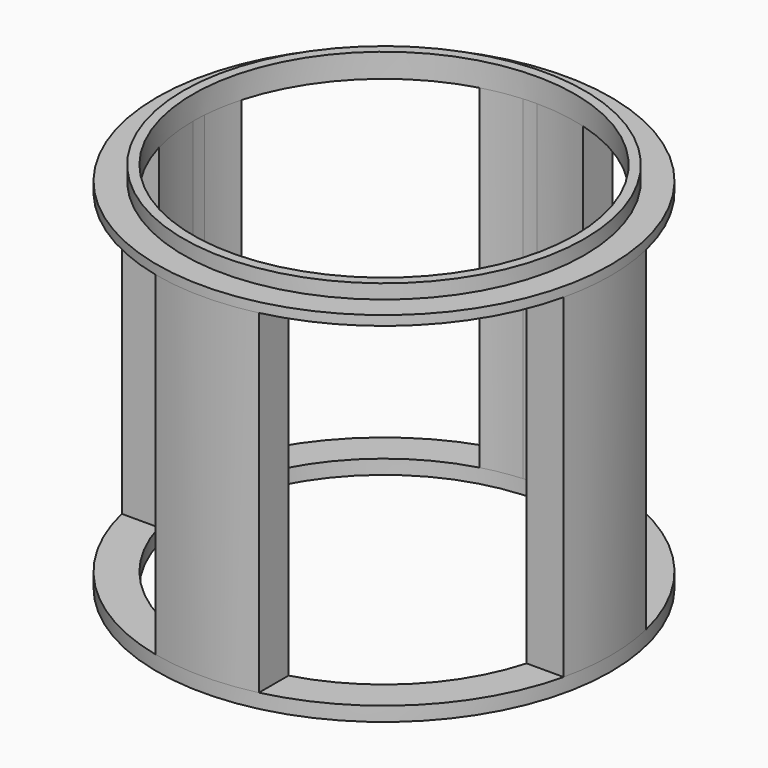
from build123d import *

# Parameters (mm, degrees)
F0_R     = 47.5
F0_R_2   = 40
F1_DEPTH = 3
F3_DEPTH = 70
F4_R     = 47.5
F4_R_2   = 40
F5_DEPTH = 2
F6_R     = 42
F6_R_2   = 40
F7_DEPTH = 3


# Not quite as in the source:
# - after a boolean that leaves OpenCascade's solid faulty, fix() repairs it


with BuildPart() as f1:
    # F0 (on Top) → F1 (new body)
    with BuildSketch(Plane.XY):
        Circle(F0_R)
        Circle(F0_R_2, mode=Mode.SUBTRACT)
    extrude(amount=F1_DEPTH)

    # F2 (on face) → F3 (join)
    with BuildSketch(Plane.XY.offset(3)):
        with BuildLine():
            Line((10.811338, 38.511232), (10.811338, 46.25327))
            ThreePointArc((10.811338, 46.25327), (0, 47.5), (-10.811338, 46.25327))
            Line((-10.811338, 46.25327), (-10.811338, 38.511232))
            ThreePointArc((-10.811338, 38.511232), (-6.865711, 39.40637), (-2.849842, 39.898351))
            ThreePointArc((-2.849842, 39.898351), (-1.425827, 39.97458), (0, 40))
            ThreePointArc((0, 40), (5.456681, 39.62606), (10.811338, 38.511232))
        make_face()
        with BuildLine():
            ThreePointArc((-39.898351, 2.849838), (-39.406371, 6.865709), (-38.511232, 10.811338))
            Line((-38.511232, 10.811338), (-46.25327, 10.811338))
            ThreePointArc((-46.25327, 10.811338), (-47.5, 0), (-46.25327, -10.811338))
            Line((-46.25327, -10.811338), (-38.511232, -10.811338))
            ThreePointArc((-38.511232, -10.811338), (-39.62606, -5.456681), (-40, 0))
            ThreePointArc((-40, 0), (-39.97458, 1.425825), (-39.898351, 2.849838))
        make_face()
        with BuildLine():
            Line((-10.811338, -38.511232), (-10.811338, -46.25327))
            ThreePointArc((-10.811338, -46.25327), (0, -47.5), (10.811338, -46.25327))
            Line((10.811338, -46.25327), (10.811338, -38.511232))
            ThreePointArc((10.811338, -38.511232), (5.456681, -39.62606), (0, -40))
            ThreePointArc((0, -40), (-5.456681, -39.62606), (-10.811338, -38.511232))
        make_face()
        with BuildLine():
            ThreePointArc((40, 0), (39.62606, -5.456681), (38.511232, -10.811338))
            Line((38.511232, -10.811338), (46.25327, -10.811338))
            ThreePointArc((46.25327, -10.811338), (47.5, 0), (46.25327, 10.811338))
            Line((46.25327, 10.811338), (38.511232, 10.811338))
            ThreePointArc((38.511232, 10.811338), (39.62606, 5.456681), (40, 0))
        make_face()
    extrude(amount=F3_DEPTH)

    add(f1.part.fix(), mode=Mode.REPLACE)

    # F4 (on face) → F5 (join)
    with BuildSketch(Plane.XY.offset(73)):
        Circle(F4_R)
        Circle(F4_R_2, mode=Mode.SUBTRACT)
    extrude(amount=F5_DEPTH)

    # F6 (on face) → F7 (join)
    with BuildSketch(Plane.XY.offset(75)):
        Circle(F6_R)
        Circle(F6_R_2, mode=Mode.SUBTRACT)
    extrude(amount=F7_DEPTH)


solid = f1.part
